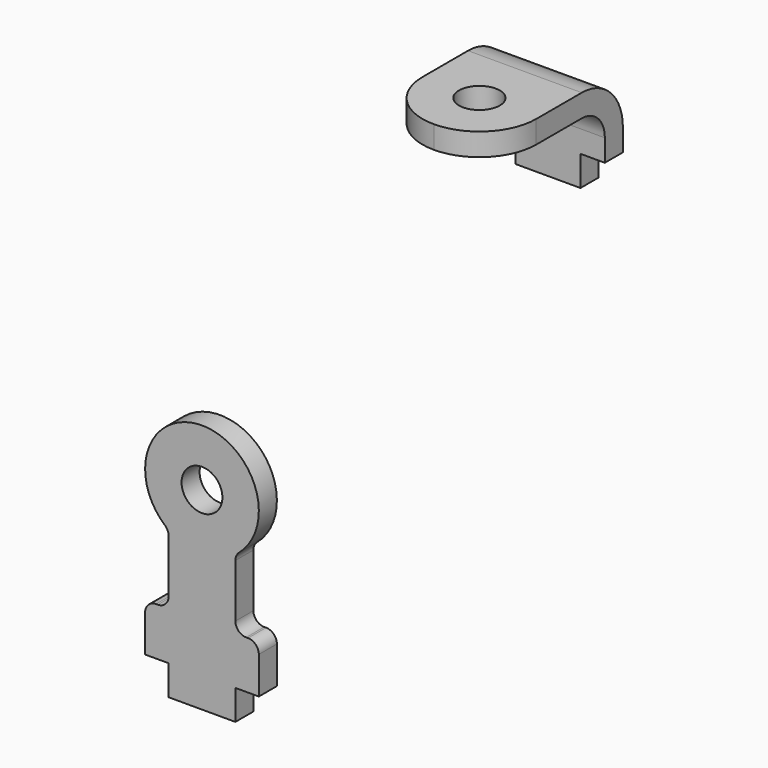
from build123d import *

# Parameters (mm, degrees)
F0_R     = 2.873
F1_DEPTH = 3.175
F3_DEPTH = 16
F4_W     = 3.429
F4_H     = 4.2418
F5_DEPTH = 25.4
F6_R     = 2.873
F7_DEPTH = 3.175


with BuildPart() as f1:
    # F0 (on Front) → F1 (new body)
    with BuildSketch(Plane.XZ):
        with BuildLine():
            ThreePointArc((-5.2068974255, -6.0735672549), (-4.831756613, -6.587290456), (-4.699, -7.2093980338))
            Line((-4.699, -7.2093980338), (-4.699, -14.7173892691))
            ThreePointArc((-4.699, -14.7173892691), (-5.1453692655, -15.7950200036), (-6.223, -16.2413892691))
            Line((-6.223, -16.2413892691), (-6.476, -16.2413892691))
            ThreePointArc((-6.476, -16.2413892691), (-7.5536307345, -16.6877585345), (-8, -17.7653892691))
            Line((-8, -17.7653892691), (-8, -22.9887201977))
            Line((-8, -22.9887201977), (-4.699, -22.9887201977))
            Line((-4.699, -22.9887201977), (-4.699, -27.2051201977))
            Line((-4.699, -27.2051201977), (0, -27.2051201977))
            Line((0, -27.2051201977), (4.699, -27.2051201977))
            Line((4.699, -27.2051201977), (4.699, -22.9887201977))
            Line((4.699, -22.9887201977), (8, -22.9887201977))
            Line((8, -22.9887201977), (8, -17.7653892691))
            ThreePointArc((8, -17.7653892691), (7.5536307345, -16.6877585345), (6.476, -16.2413892691))
            Line((6.476, -16.2413892691), (6.223, -16.2413892691))
            ThreePointArc((6.223, -16.2413892691), (5.1453692655, -15.7950200036), (4.699, -14.7173892691))
            Line((4.699, -14.7173892691), (4.699, -7.2093980338))
            ThreePointArc((4.699, -7.2093980338), (4.831756613, -6.587290456), (5.2068974255, -6.0735672549))
            ThreePointArc((5.2068974255, -6.0735672549), (0, 8), (-5.2068974255, -6.0735672549))
        make_face()
        Circle(F0_R, mode=Mode.SUBTRACT)
    extrude(amount=F1_DEPTH)


with BuildPart() as f3:
    # F2 (on Right) → F3 (new body)
    with BuildSketch(Plane.YZ):
        with BuildLine():
            Line((47.6821554806, 20.8151274502), (50.8571554806, 20.8151274502))
            Line((50.8571554806, 20.8151274502), (50.8571554806, 28.1511274502))
            ThreePointArc((50.8571554806, 28.1511274502), (48.7369014696, 33.2698734392), (43.6181554806, 35.3901274502))
            Line((43.6181554806, 35.3901274502), (27.6181554806, 35.3901274502))
            Line((27.6181554806, 35.3901274502), (27.6181554806, 32.2151274502))
            Line((27.6181554806, 32.2151274502), (43.6181554806, 32.2151274502))
            ThreePointArc((43.6181554806, 32.2151274502), (46.4918374394, 31.024809409), (47.6821554806, 28.1511274502))
            Line((47.6821554806, 28.1511274502), (47.6821554806, 20.8151274502))
        make_face()
    extrude(amount=F3_DEPTH)

    # F4 (on face) → F5 (cut)
    with BuildSketch(Plane(origin=(0, 50.8571554806, 0), x_dir=(-1, 0, 0), z_dir=(0, 1, 0))):
        with Locations((-14.2855, 22.9360274502)):
            Rectangle(F4_W, F4_H)
        with Locations((-1.7145, 22.9360274502)):
            Rectangle(F4_W, F4_H)
    extrude(amount=-F5_DEPTH, mode=Mode.SUBTRACT)

    # F6 (on face) → F7 (cut, through all)
    with BuildSketch(Plane.XY.offset(35.3901274502)):
        with BuildLine():
            Line((0, 27.6181554806), (8, 27.6181554806))
            ThreePointArc((8, 27.6181554806), (2.3431457505, 29.9613012311), (0, 35.6181554806))
            Line((0, 35.6181554806), (0, 27.6181554806))
        make_face()
        with BuildLine():
            Line((16, 27.6181554806), (16, 35.6181554806))
            ThreePointArc((16, 35.6181554806), (13.6568542495, 29.9613012311), (8, 27.6181554806))
            Line((8, 27.6181554806), (16, 27.6181554806))
        make_face()
        with Locations((8, 35.6181554806)):
            Circle(F6_R)
    extrude(amount=-F7_DEPTH, mode=Mode.SUBTRACT)


solid = Compound([f1.part, f3.part])
